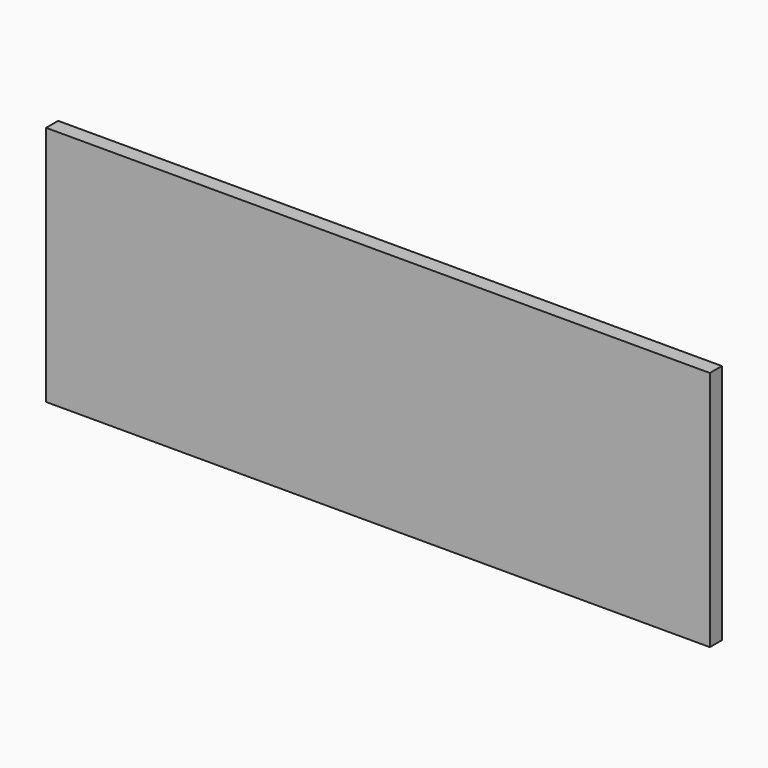
from build123d import *

# Parameters (mm, degrees)
F0_W     = 558.8
F0_H     = 203.2
F1_DEPTH = 12.7


# Not quite as in the source:
# - a length typed as a fraction of an inch, garbled in the dataset ("3 / 203.2 mm" for 3/8 in), is restored


with BuildPart() as f1:
    # F0 (on Front) → F1 (new body)
    with BuildSketch(Plane.XZ):
        Rectangle(F0_W, F0_H)
    extrude(amount=F1_DEPTH)


solid = f1.part
